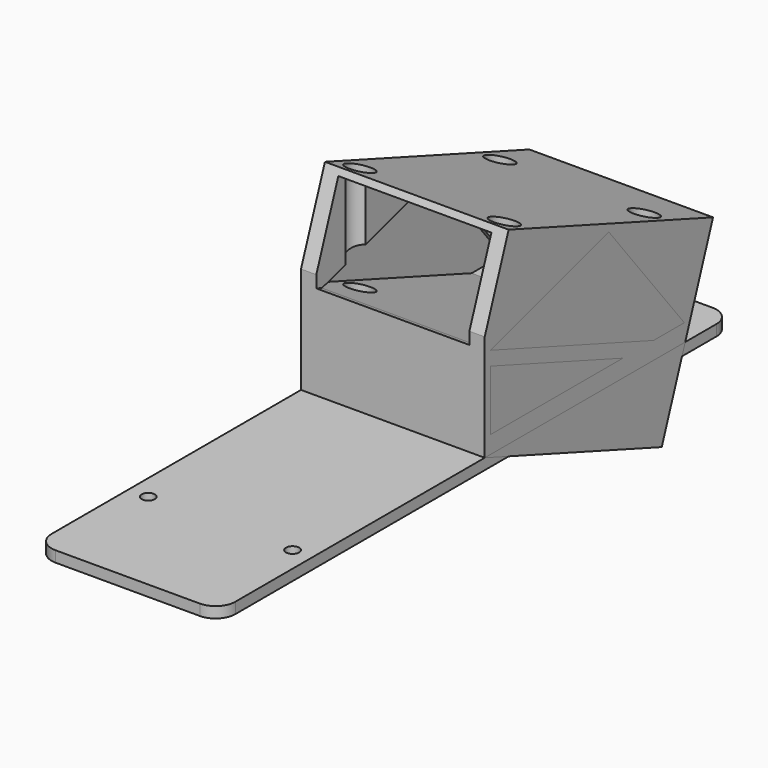
from build123d import *

# Parameters (mm, degrees)
F0_R           = 1.5
F1_DEPTH       = 2.5
F3_DEPTH       = 21
F3_DEPTH_BACK  = 21
F5_DEPTH       = 42
F6_DEPTH       = 3.5
F8_DEPTH       = 3.5
F9_R           = 9
F10_DEPTH      = 5
F11_W          = 35
F11_H          = 2.6059500945
F12_DEPTH      = 5
F13_R          = 1.5
F14_DEPTH      = 5
F15_R          = 3
F16_DEPTH      = 1.5
F16_DEPTH_BACK = 40
F18_DEPTH      = 0.4
F20_DEPTH      = 0.4
F21_R          = 9
F22_DEPTH      = 0.4
F24_DEPTH      = 21
F24_DEPTH_BACK = 21
F25_START      = 20.6
F25_DEPTH      = 0.4
F26_START      = -20.6
F26_DEPTH      = 0.4


with BuildPart() as f1:
    # F0 (on Top) → F1 (new body)
    with BuildSketch(Plane.XY):
        with BuildLine():
            Line((-21, 87.25), (-21, 71.75))
            Line((-21, 71.75), (-21, -44.25))
            Line((-21, -44.25), (-21, -50.25))
            ThreePointArc((-21, -50.25), (-19.6819805153, -53.4319805153), (-16.5, -54.75))
            Line((-16.5, -54.75), (16.5, -54.75))
            ThreePointArc((16.5, -54.75), (19.6819805153, -53.4319805153), (21, -50.25))
            Line((21, -50.25), (21, -44.25))
            Line((21, -44.25), (21, 72.25))
            Line((21, 72.25), (21, 87.25))
            ThreePointArc((21, 87.25), (19.6819805153, 90.4319805153), (16.5, 91.75))
            Line((16.5, 91.75), (-16.5, 91.75))
            ThreePointArc((-16.5, 91.75), (-19.6819805153, 90.4319805153), (-21, 87.25))
        make_face()
        with Locations((-16.5, -28.25)):
            Circle(F0_R, mode=Mode.SUBTRACT)
        with Locations((16.5, -28.25)):
            Circle(F0_R, mode=Mode.SUBTRACT)
        with Locations((-16.5, 32.25)):
            Circle(F0_R, mode=Mode.SUBTRACT)
        with Locations((-16.5, 72.25)):
            Circle(F0_R, mode=Mode.SUBTRACT)
        with Locations((16.5, 32.25)):
            Circle(F0_R, mode=Mode.SUBTRACT)
        with Locations((16.5, 72.25)):
            Circle(F0_R, mode=Mode.SUBTRACT)
    extrude(amount=F1_DEPTH)


with BuildPart() as f3:
    # F2 (on Right) → F3 (new body, two sides)
    with BuildSketch(Plane.YZ) as f3_sk:
        Polygon((78.3229025326, 2.5), (79.579607227, 5.9527677707), (86.2832020362, 24.3707431381), (27.8726022217, 45.6304628362), (21.0342344073, 26.8422016804), (21.0342344073, 2.5), (22.6342344073, 2.5), align=None)
        Polygon((22.6342344073, 6.5), (22.6342344073, 26.6791884562), (28.7905969872, 43.5936556304), (84.2324616136, 23.4144671741), (78.0760990337, 6.5), align=None, mode=Mode.SUBTRACT)
    extrude(amount=F3_DEPTH)
    extrude(f3_sk.sketch, amount=-F3_DEPTH_BACK)

    # F4 (on face) → F5 (join)
    with BuildSketch(Plane.YZ.offset(21)):
        Polygon((60.5332726327, 6.5), (69.3046858332, 6.5), (22.6342344073, 23.4866551388), (22.6342344073, 20.2941218214), align=None)
    extrude(amount=-F5_DEPTH)

    # F4 (on face) → F6 (join)
    with BuildSketch(Plane.YZ.offset(21)):
        Polygon((56.5115293004, 33.5040614023), (78.0760990337, 6.5), (84.2324616136, 23.4144671741), align=None)
        Polygon((22.6342344073, 26.6791884562), (22.6342344073, 23.4866551388), (56.5115293004, 33.5040614023), (28.7905969872, 43.5936556304), align=None)
    extrude(amount=-F6_DEPTH)

    # F7 (on face) → F8 (join)
    with BuildSketch(Plane(origin=(-21, 0, 0), x_dir=(0, -1, 0), z_dir=(-1, 0, 0))):
        Polygon((-78.0760990337, 6.5), (-56.5115293004, 33.5040614023), (-84.2324616136, 23.4144671741), align=None)
        Polygon((-56.5115293004, 33.5040614023), (-22.6342344073, 23.4866551388), (-22.6342344073, 26.6791884562), (-28.7905969872, 43.5936556304), align=None)
    extrude(amount=-F8_DEPTH)

    # F9 (on face) → F10 (cut)
    with BuildSketch(Plane(origin=(0, 68.3573788812, -24.8800512052), x_dir=(-1, 0, 0), z_dir=(0, 0.9396926208, -0.3420201433))):
        with Locations((0, 41.8116006169)):
            Circle(F9_R)
    extrude(amount=-F10_DEPTH, mode=Mode.SUBTRACT)

    # F11 (on face) → F12 (cut)
    with BuildSketch(Plane(origin=(0, 9.9467790667, -3.6203315071), x_dir=(1, 0, 0), z_dir=(0, -0.9396926208, 0.3420201433))):
        Polygon((-17.5, 50.8116006169), (-17.5, 32.8116006169), (-17.5, 32.4175507114), (17.5, 32.4175507114), (17.5, 32.8116006169), (17.5, 50.8116006169), align=None)
        with Locations((0, 31.1145756642)):
            Rectangle(F11_W, F11_H)
    extrude(amount=-F12_DEPTH, mode=Mode.SUBTRACT)

    # F13 (on face) → F14 (cut)
    with BuildSketch(Plane.XY.offset(6.5)):
        with Locations((-16.5, 32.25)):
            Circle(F13_R)
        with Locations((16.5, 32.25)):
            Circle(F13_R)
        with Locations((16.5, 72.25)):
            Circle(F13_R)
        with Locations((-16.5, 72.25)):
            Circle(F13_R)
    extrude(amount=-F14_DEPTH, mode=Mode.SUBTRACT)

    # F15 (on face) → F16 (cut, two sides)
    with BuildSketch(Plane.XY.offset(6.5)) as f16_sk:
        with Locations((-16.5, 32.25)):
            Circle(F15_R)
        with Locations((16.5, 32.25)):
            Circle(F15_R)
        with Locations((16.5, 72.25)):
            Circle(F15_R)
        with Locations((-16.5, 72.25)):
            Circle(F15_R)
    extrude(amount=-F16_DEPTH, mode=Mode.SUBTRACT)
    extrude(f16_sk.sketch, amount=F16_DEPTH_BACK, mode=Mode.SUBTRACT)


with BuildPart() as f18:
    # F17 (on face) → F18 (new body)
    with BuildSketch(Plane.YZ.offset(21)):
        Polygon((22.6342344073, 23.4866551388), (69.3046858332, 6.5), (78.0760990337, 6.5), (56.5115293004, 33.5040614023), align=None)
    extrude(amount=-F18_DEPTH)


with BuildPart() as f18b:
    # F17 (on face) → F18, piece 2 (new body)
    with BuildSketch(Plane.YZ.offset(21)):
        Polygon((22.6342344073, 6.5), (60.5332726327, 6.5), (22.6342344073, 20.2941218214), align=None)
    extrude(amount=-F18_DEPTH)


with BuildPart() as f20:
    # F19 (on face) → F20 (new body)
    with BuildSketch(Plane(origin=(-21, 0, 0), x_dir=(0, -1, 0), z_dir=(-1, 0, 0))):
        Polygon((-69.3046858332, 6.5), (-22.6342344073, 23.4866551388), (-56.5115293004, 33.5040614023), (-78.0760990337, 6.5), align=None)
    extrude(amount=-F20_DEPTH)


with BuildPart() as f20b:
    # F19 (on face) → F20, piece 2 (new body)
    with BuildSketch(Plane(origin=(-21, 0, 0), x_dir=(0, -1, 0), z_dir=(-1, 0, 0))):
        Polygon((-22.6342344073, 20.2941218214), (-60.5332726327, 6.5), (-22.6342344073, 6.5), align=None)
    extrude(amount=-F20_DEPTH)


with BuildPart() as f22:
    # F21 (on face) → F22 (new body)
    with BuildSketch(Plane(origin=(0, 68.3573788812, -24.8800512052), x_dir=(-1, 0, 0), z_dir=(0, 0.9396926208, -0.3420201433))):
        with Locations((0, 41.8116006169)):
            Circle(F21_R)
    extrude(amount=-F22_DEPTH)


with BuildPart() as f24:
    # F23 (on Right) → F24 (new body, two sides)
    with BuildSketch(Plane.YZ) as f24_sk:
        Polygon((71.6214014055, -15.9122230232), (78.3229025326, 2.5), (77.8972314236, 2.5), (71.2455243572, -15.7754149659), align=None)
    extrude(amount=F24_DEPTH)
    extrude(f24_sk.sketch, amount=-F24_DEPTH_BACK)

    # F23 (on Right) → F25 (join)
    with BuildSketch(Plane.YZ.offset(F25_START)):
        Polygon((71.2455243572, -15.7754149659), (77.8972314236, 2.5), (21.0342344073, 2.5), align=None)
    extrude(amount=F25_DEPTH)

    # F23 (on Right) → F26 (join)
    with BuildSketch(Plane.YZ.offset(F26_START)):
        Polygon((71.2455243572, -15.7754149659), (77.8972314236, 2.5), (21.0342344073, 2.5), align=None)
    extrude(amount=-F26_DEPTH)


solid = Compound([f1.part, f3.part, f18.part, f18b.part, f20.part, f20b.part, f22.part, f24.part])
